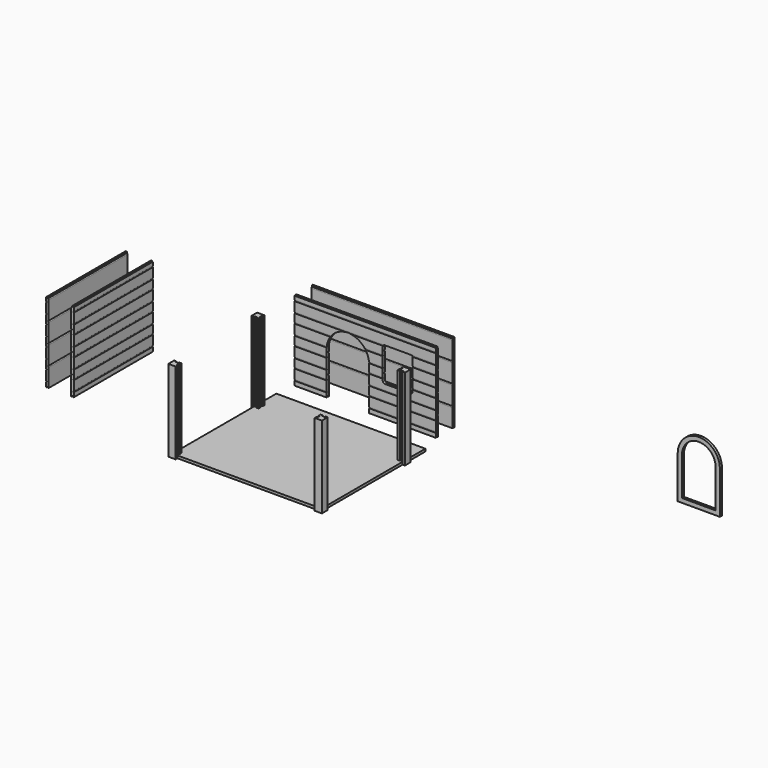
from build123d import *

# Parameters (mm, degrees)
F0_W      = 700
F0_H      = 610
F1_DEPTH  = 12
F3_DEPTH  = 384
F4_START  = -12
F4_DEPTH  = 372
F6_DEPTH  = 463.5
F8_DEPTH  = 663.5
F9_W      = 200
F9_H      = 85
F10_DEPTH = 12.5
F11_DEPTH = 12


with BuildPart() as f1:
    # F0 (on Top) → F1 (new body)
    with BuildSketch(Plane.XY):
        with Locations((0, 55)):
            Rectangle(F0_W, F0_H)
    extrude(amount=F1_DEPTH)


with BuildPart() as f3:
    # F2 (on face) → F3 (new body)
    with BuildSketch(Plane(origin=(0, 0, 0), x_dir=(1, 0, 0), z_dir=(0, 0, -1))):
        Polygon((-350, 226.75), (-350, 231.75), (-350, 250), (-331.75, 250), (-326.75, 250), (-326.75, 260.75), (-360.75, 260.75), (-360.75, 226.75), align=None)
    extrude(amount=-F3_DEPTH)

    # F2 (on face) → F4, piece 2 (join)
    with BuildSketch(Plane(origin=(0, 0, 0), x_dir=(1, 0, 0), z_dir=(0, 0, -1)).offset(F4_START)):
        Polygon((-337.5, 226.75), (-326.75, 226.75), (-326.75, 237.5), (-331.75, 237.5), (-331.75, 250), (-350, 250), (-350, 231.75), (-337.5, 231.75), align=None)
    extrude(amount=-F4_DEPTH)


with BuildPart() as f3b:
    # F2 (on face) → F3, piece 2 (new body)
    with BuildSketch(Plane(origin=(0, 0, 0), x_dir=(1, 0, 0), z_dir=(0, 0, -1))):
        Polygon((-350, -231.75), (-350, -226.75), (-360.75, -226.75), (-360.75, -260.75), (-350, -260.75), (-350, -250), align=None)
    extrude(amount=-F3_DEPTH)

    # F2 (on face) → F4, piece 4 (join)
    with BuildSketch(Plane(origin=(0, 0, 0), x_dir=(1, 0, 0), z_dir=(0, 0, -1)).offset(F4_START)):
        Polygon((-337.5, -231.75), (-350, -231.75), (-350, -250), (-350, -260.75), (-326.75, -260.75), (-326.75, -250), (-331.75, -250), (-331.75, -237.5), (-326.75, -237.5), (-326.75, -226.75), (-337.5, -226.75), align=None)
    extrude(amount=-F4_DEPTH)


with BuildPart() as f3c:
    # F2 (on face) → F3, piece 3 (new body)
    with BuildSketch(Plane(origin=(0, 0, 0), x_dir=(1, 0, 0), z_dir=(0, 0, -1))):
        Polygon((326.75, 260.75), (326.75, 250), (331.75, 250), (350, 250), (350, 231.75), (350, 226.75), (360.75, 226.75), (360.75, 260.75), align=None)
    extrude(amount=-F3_DEPTH)

    # F2 (on face) → F4 (join)
    with BuildSketch(Plane(origin=(0, 0, 0), x_dir=(1, 0, 0), z_dir=(0, 0, -1)).offset(F4_START)):
        Polygon((350, 250), (331.75, 250), (331.75, 237.5), (326.75, 237.5), (326.75, 226.75), (337.5, 226.75), (337.5, 231.75), (350, 231.75), align=None)
    extrude(amount=-F4_DEPTH)


with BuildPart() as f3d:
    # F2 (on face) → F3, piece 4 (new body)
    with BuildSketch(Plane(origin=(0, 0, 0), x_dir=(1, 0, 0), z_dir=(0, 0, -1))):
        Polygon((360.75, -226.75), (350, -226.75), (350, -231.75), (350, -250), (350, -260.75), (360.75, -260.75), align=None)
    extrude(amount=-F3_DEPTH)

    # F2 (on face) → F4, piece 3 (join)
    with BuildSketch(Plane(origin=(0, 0, 0), x_dir=(1, 0, 0), z_dir=(0, 0, -1)).offset(F4_START)):
        Polygon((326.75, -260.75), (350, -260.75), (350, -250), (350, -231.75), (337.5, -231.75), (337.5, -226.75), (326.75, -226.75), (326.75, -237.5), (331.75, -237.5), (331.75, -250), (326.75, -250), align=None)
    extrude(amount=-F4_DEPTH)


with BuildPart() as f6:
    # F5 (on face) → F6 (new body)
    with BuildSketch(Plane.XZ.offset(-231.75)):
        with BuildLine():
            Line((-836.1184597015, 267.9065500498), (-836.1184597015, 263.9065500498))
            Line((-836.1184597015, 263.9065500498), (-836.3684597015, 263.9065500498))
            ThreePointArc((-836.3684597015, 263.9065500498), (-839.1968868263, 262.7349771745), (-840.3684597015, 259.9065500498))
            Line((-840.3684597015, 259.9065500498), (-840.3684597015, 174.9065500498))
            Line((-840.3684597015, 174.9065500498), (-836.1184597015, 174.9065500498))
            Line((-836.1184597015, 174.9065500498), (-836.1184597015, 170.9065500498))
            Line((-836.1184597015, 170.9065500498), (-836.3684597015, 170.9065500498))
            ThreePointArc((-836.3684597015, 170.9065500498), (-839.1968868263, 169.7349771745), (-840.3684597015, 166.9065500498))
            Line((-840.3684597015, 166.9065500498), (-840.3684597015, 81.9065500498))
            Line((-840.3684597015, 81.9065500498), (-836.1184597015, 81.9065500498))
            Line((-836.1184597015, 81.9065500498), (-836.1184597015, 84.9065500498))
            Line((-836.1184597015, 84.9065500498), (-832.1184597015, 84.9065500498))
            Line((-832.1184597015, 84.9065500498), (-832.1184597015, 81.9065500498))
            Line((-832.1184597015, 81.9065500498), (-827.8684597015, 81.9065500498))
            Line((-827.8684597015, 81.9065500498), (-827.8684597015, 102.4065500498))
            ThreePointArc((-827.8684597015, 102.4065500498), (-830.3684597015, 104.9065500498), (-827.8684597015, 107.4065500498))
            Line((-827.8684597015, 107.4065500498), (-827.8684597015, 129.9065500498))
            Line((-827.8684597015, 129.9065500498), (-827.8684597015, 152.4065500498))
            ThreePointArc((-827.8684597015, 152.4065500498), (-830.3684597015, 154.9065500498), (-827.8684597015, 157.4065500498))
            Line((-827.8684597015, 157.4065500498), (-827.8684597015, 174.9065500498))
            Line((-827.8684597015, 174.9065500498), (-827.8684597015, 195.4065500498))
            ThreePointArc((-827.8684597015, 195.4065500498), (-830.3684597015, 197.9065500498), (-827.8684597015, 200.4065500498))
            Line((-827.8684597015, 200.4065500498), (-827.8684597015, 222.9065500498))
            Line((-827.8684597015, 222.9065500498), (-827.8684597015, 245.4065500498))
            ThreePointArc((-827.8684597015, 245.4065500498), (-830.3684597015, 247.9065500498), (-827.8684597015, 250.4065500498))
            Line((-827.8684597015, 250.4065500498), (-827.8684597015, 267.9065500498))
            Line((-827.8684597015, 267.9065500498), (-827.8684597015, 288.4065500498))
            ThreePointArc((-827.8684597015, 288.4065500498), (-830.3684597015, 290.9065500498), (-827.8684597015, 293.4065500498))
            Line((-827.8684597015, 293.4065500498), (-827.8684597015, 315.9065500498))
            Line((-827.8684597015, 315.9065500498), (-827.8684597015, 338.4065500498))
            ThreePointArc((-827.8684597015, 338.4065500498), (-830.3684597015, 340.9065500498), (-827.8684597015, 343.4065500498))
            Line((-827.8684597015, 343.4065500498), (-827.8684597015, 360.9065500498))
            Line((-827.8684597015, 360.9065500498), (-827.8684597015, 381.4065500498))
            ThreePointArc((-827.8684597015, 381.4065500498), (-830.3684597015, 383.9065500498), (-827.8684597015, 386.4065500498))
            Line((-827.8684597015, 386.4065500498), (-827.8684597015, 408.9065500498))
            Line((-827.8684597015, 408.9065500498), (-827.8684597015, 431.4065500498))
            ThreePointArc((-827.8684597015, 431.4065500498), (-830.3684597015, 433.9065500498), (-827.8684597015, 436.4065500498))
            Line((-827.8684597015, 436.4065500498), (-827.8684597015, 453.9065500498))
            Line((-827.8684597015, 453.9065500498), (-832.1184597015, 453.9065500498))
            Line((-832.1184597015, 453.9065500498), (-832.1184597015, 456.9065500498))
            Line((-832.1184597015, 456.9065500498), (-834.1184597015, 456.9065500498))
            Line((-834.1184597015, 456.9065500498), (-836.1184597015, 456.9065500498))
            Line((-836.1184597015, 456.9065500498), (-836.1184597015, 449.9065500498))
            Line((-836.1184597015, 449.9065500498), (-836.3684597015, 449.9065500498))
            ThreePointArc((-836.3684597015, 449.9065500498), (-839.1968868263, 448.7349771745), (-840.3684597015, 445.9065500498))
            Line((-840.3684597015, 445.9065500498), (-840.3684597015, 360.9065500498))
            Line((-840.3684597015, 360.9065500498), (-836.1184597015, 360.9065500498))
            Line((-836.1184597015, 360.9065500498), (-836.1184597015, 356.9065500498))
            Line((-836.1184597015, 356.9065500498), (-836.3684597015, 356.9065500498))
            ThreePointArc((-836.3684597015, 356.9065500498), (-839.1968868263, 355.7349771745), (-840.3684597015, 352.9065500498))
            Line((-840.3684597015, 352.9065500498), (-840.3684597015, 267.9065500498))
            Line((-840.3684597015, 267.9065500498), (-836.1184597015, 267.9065500498))
        make_face()
    extrude(amount=F6_DEPTH)


with BuildPart() as f6b:
    # F5 (on face) → F6, piece 2 (new body)
    with BuildSketch(Plane.XZ.offset(-231.75)):
        with BuildLine():
            Line((-949.6443090439, 170.9065500498), (-949.8943090439, 170.9065500498))
            Line((-949.8943090439, 170.9065500498), (-949.8943090439, 174.9065500498))
            Line((-949.8943090439, 174.9065500498), (-945.6443090439, 174.9065500498))
            Line((-945.6443090439, 174.9065500498), (-945.6443090439, 259.9065500498))
            ThreePointArc((-945.6443090439, 259.9065500498), (-946.8158819191, 262.7349771745), (-949.6443090439, 263.9065500498))
            Line((-949.6443090439, 263.9065500498), (-949.8943090439, 263.9065500498))
            Line((-949.8943090439, 263.9065500498), (-949.8943090439, 267.9065500498))
            Line((-949.8943090439, 267.9065500498), (-945.6443090439, 267.9065500498))
            Line((-945.6443090439, 267.9065500498), (-945.6443090439, 352.9065500498))
            ThreePointArc((-945.6443090439, 352.9065500498), (-946.8158819191, 355.7349771745), (-949.6443090439, 356.9065500498))
            Line((-949.6443090439, 356.9065500498), (-949.8943090439, 356.9065500498))
            Line((-949.8943090439, 356.9065500498), (-949.8943090439, 360.9065500498))
            Line((-949.8943090439, 360.9065500498), (-945.6443090439, 360.9065500498))
            Line((-945.6443090439, 360.9065500498), (-945.6443090439, 445.9065500498))
            ThreePointArc((-945.6443090439, 445.9065500498), (-946.8158819191, 448.7349771745), (-949.6443090439, 449.9065500498))
            Line((-949.6443090439, 449.9065500498), (-949.8943090439, 449.9065500498))
            Line((-949.8943090439, 449.9065500498), (-949.8943090439, 456.9065500498))
            Line((-949.8943090439, 456.9065500498), (-951.8943090439, 456.9065500498))
            Line((-951.8943090439, 456.9065500498), (-953.8943090439, 456.9065500498))
            Line((-953.8943090439, 456.9065500498), (-953.8943090439, 453.9065500498))
            Line((-953.8943090439, 453.9065500498), (-958.1443090439, 453.9065500498))
            Line((-958.1443090439, 453.9065500498), (-958.1443090439, 436.4065500498))
            ThreePointArc((-958.1443090439, 436.4065500498), (-955.6443090439, 433.9065500498), (-958.1443090439, 431.4065500498))
            Line((-958.1443090439, 431.4065500498), (-958.1443090439, 408.9065500498))
            Line((-958.1443090439, 408.9065500498), (-958.1443090439, 386.4065500498))
            ThreePointArc((-958.1443090439, 386.4065500498), (-955.6443090439, 383.9065500498), (-958.1443090439, 381.4065500498))
            Line((-958.1443090439, 381.4065500498), (-958.1443090439, 360.9065500498))
            Line((-958.1443090439, 360.9065500498), (-958.1443090439, 343.4065500498))
            ThreePointArc((-958.1443090439, 343.4065500498), (-955.6443090439, 340.9065500498), (-958.1443090439, 338.4065500498))
            Line((-958.1443090439, 338.4065500498), (-958.1443090439, 315.9065500498))
            Line((-958.1443090439, 315.9065500498), (-958.1443090439, 293.4065500498))
            ThreePointArc((-958.1443090439, 293.4065500498), (-955.6443090439, 290.9065500498), (-958.1443090439, 288.4065500498))
            Line((-958.1443090439, 288.4065500498), (-958.1443090439, 267.9065500498))
            Line((-958.1443090439, 267.9065500498), (-958.1443090439, 250.4065500498))
            ThreePointArc((-958.1443090439, 250.4065500498), (-955.6443090439, 247.9065500498), (-958.1443090439, 245.4065500498))
            Line((-958.1443090439, 245.4065500498), (-958.1443090439, 222.9065500498))
            Line((-958.1443090439, 222.9065500498), (-958.1443090439, 200.4065500498))
            ThreePointArc((-958.1443090439, 200.4065500498), (-955.6443090439, 197.9065500498), (-958.1443090439, 195.4065500498))
            Line((-958.1443090439, 195.4065500498), (-958.1443090439, 174.9065500498))
            Line((-958.1443090439, 174.9065500498), (-958.1443090439, 157.4065500498))
            ThreePointArc((-958.1443090439, 157.4065500498), (-955.6443090439, 154.9065500498), (-958.1443090439, 152.4065500498))
            Line((-958.1443090439, 152.4065500498), (-958.1443090439, 129.9065500498))
            Line((-958.1443090439, 129.9065500498), (-958.1443090439, 107.4065500498))
            ThreePointArc((-958.1443090439, 107.4065500498), (-955.6443090439, 104.9065500498), (-958.1443090439, 102.4065500498))
            Line((-958.1443090439, 102.4065500498), (-958.1443090439, 81.9065500498))
            Line((-958.1443090439, 81.9065500498), (-953.8943090439, 81.9065500498))
            Line((-953.8943090439, 81.9065500498), (-953.8943090439, 84.9065500498))
            Line((-953.8943090439, 84.9065500498), (-949.8943090439, 84.9065500498))
            Line((-949.8943090439, 84.9065500498), (-949.8943090439, 81.9065500498))
            Line((-949.8943090439, 81.9065500498), (-945.6443090439, 81.9065500498))
            Line((-945.6443090439, 81.9065500498), (-945.6443090439, 166.9065500498))
            ThreePointArc((-945.6443090439, 166.9065500498), (-946.8158819191, 169.7349771745), (-949.6443090439, 170.9065500498))
        make_face()
    extrude(amount=F6_DEPTH)


with BuildPart() as f8:
    # F7 (on face) → F8 (new body)
    with BuildSketch(Plane(origin=(331.75, 0, 0), x_dir=(0, -1, 0), z_dir=(-1, 0, 0))):
        with BuildLine():
            Line((-546.5363952824, 104.9655441736), (-546.7863952824, 104.9655441736))
            Line((-546.7863952824, 104.9655441736), (-546.7863952824, 108.9655441736))
            Line((-546.7863952824, 108.9655441736), (-542.5363952824, 108.9655441736))
            Line((-542.5363952824, 108.9655441736), (-542.5363952824, 193.9655441736))
            ThreePointArc((-542.5363952824, 193.9655441736), (-543.7079681576, 196.7939712984), (-546.5363952824, 197.9655441736))
            Line((-546.5363952824, 197.9655441736), (-546.7863952824, 197.9655441736))
            Line((-546.7863952824, 197.9655441736), (-546.7863952824, 201.9655441736))
            Line((-546.7863952824, 201.9655441736), (-542.5363952824, 201.9655441736))
            Line((-542.5363952824, 201.9655441736), (-542.5363952824, 286.9655441736))
            ThreePointArc((-542.5363952824, 286.9655441736), (-543.7079681576, 289.7939712984), (-546.5363952824, 290.9655441736))
            Line((-546.5363952824, 290.9655441736), (-546.7863952824, 290.9655441736))
            Line((-546.7863952824, 290.9655441736), (-546.7863952824, 294.9655441736))
            Line((-546.7863952824, 294.9655441736), (-542.5363952824, 294.9655441736))
            Line((-542.5363952824, 294.9655441736), (-542.5363952824, 379.9655441736))
            ThreePointArc((-542.5363952824, 379.9655441736), (-543.7079681576, 382.7939712984), (-546.5363952824, 383.9655441736))
            Line((-546.5363952824, 383.9655441736), (-546.7863952824, 383.9655441736))
            Line((-546.7863952824, 383.9655441736), (-546.7863952824, 390.9655441736))
            Line((-546.7863952824, 390.9655441736), (-548.7863952824, 390.9655441736))
            Line((-548.7863952824, 390.9655441736), (-550.7863952824, 390.9655441736))
            Line((-550.7863952824, 390.9655441736), (-550.7863952824, 387.9655441736))
            Line((-550.7863952824, 387.9655441736), (-555.0363952824, 387.9655441736))
            Line((-555.0363952824, 387.9655441736), (-555.0363952824, 370.4655441736))
            ThreePointArc((-555.0363952824, 370.4655441736), (-552.5363952824, 367.9655441736), (-555.0363952824, 365.4655441736))
            Line((-555.0363952824, 365.4655441736), (-555.0363952824, 342.9655441736))
            Line((-555.0363952824, 342.9655441736), (-555.0363952824, 320.4655441736))
            ThreePointArc((-555.0363952824, 320.4655441736), (-552.5363952824, 317.9655441736), (-555.0363952824, 315.4655441736))
            Line((-555.0363952824, 315.4655441736), (-555.0363952824, 294.9655441736))
            Line((-555.0363952824, 294.9655441736), (-555.0363952824, 277.4655441736))
            ThreePointArc((-555.0363952824, 277.4655441736), (-552.5363952824, 274.9655441736), (-555.0363952824, 272.4655441736))
            Line((-555.0363952824, 272.4655441736), (-555.0363952824, 249.9655441736))
            Line((-555.0363952824, 249.9655441736), (-555.0363952824, 227.4655441736))
            ThreePointArc((-555.0363952824, 227.4655441736), (-552.5363952824, 224.9655441736), (-555.0363952824, 222.4655441736))
            Line((-555.0363952824, 222.4655441736), (-555.0363952824, 201.9655441736))
            Line((-555.0363952824, 201.9655441736), (-555.0363952824, 184.4655441736))
            ThreePointArc((-555.0363952824, 184.4655441736), (-552.5363952824, 181.9655441736), (-555.0363952824, 179.4655441736))
            Line((-555.0363952824, 179.4655441736), (-555.0363952824, 156.9655441736))
            Line((-555.0363952824, 156.9655441736), (-555.0363952824, 134.4655441736))
            ThreePointArc((-555.0363952824, 134.4655441736), (-552.5363952824, 131.9655441736), (-555.0363952824, 129.4655441736))
            Line((-555.0363952824, 129.4655441736), (-555.0363952824, 108.9655441736))
            Line((-555.0363952824, 108.9655441736), (-555.0363952824, 91.4655441736))
            ThreePointArc((-555.0363952824, 91.4655441736), (-552.5363952824, 88.9655441736), (-555.0363952824, 86.4655441736))
            Line((-555.0363952824, 86.4655441736), (-555.0363952824, 63.9655441736))
            Line((-555.0363952824, 63.9655441736), (-555.0363952824, 41.4655441736))
            ThreePointArc((-555.0363952824, 41.4655441736), (-552.5363952824, 38.9655441736), (-555.0363952824, 36.4655441736))
            Line((-555.0363952824, 36.4655441736), (-555.0363952824, 15.9655441736))
            Line((-555.0363952824, 15.9655441736), (-550.7863952824, 15.9655441736))
            Line((-550.7863952824, 15.9655441736), (-550.7863952824, 18.9655441736))
            Line((-550.7863952824, 18.9655441736), (-546.7863952824, 18.9655441736))
            Line((-546.7863952824, 18.9655441736), (-546.7863952824, 15.9655441736))
            Line((-546.7863952824, 15.9655441736), (-542.5363952824, 15.9655441736))
            Line((-542.5363952824, 15.9655441736), (-542.5363952824, 100.9655441736))
            ThreePointArc((-542.5363952824, 100.9655441736), (-543.7079681576, 103.7939712984), (-546.5363952824, 104.9655441736))
        make_face()
    extrude(amount=F8_DEPTH)


with BuildPart() as f8b:
    # F7 (on face) → F8, piece 2 (new body)
    with BuildSketch(Plane(origin=(331.75, 0, 0), x_dir=(0, -1, 0), z_dir=(-1, 0, 0))):
        with BuildLine():
            Line((-453.3388936809, 108.9655441736), (-453.3388936809, 104.9655441736))
            Line((-453.3388936809, 104.9655441736), (-453.5888936809, 104.9655441736))
            ThreePointArc((-453.5888936809, 104.9655441736), (-456.4173208057, 103.7939712984), (-457.5888936809, 100.9655441736))
            Line((-457.5888936809, 100.9655441736), (-457.5888936809, 15.9655441736))
            Line((-457.5888936809, 15.9655441736), (-453.3388936809, 15.9655441736))
            Line((-453.3388936809, 15.9655441736), (-453.3388936809, 18.9655441736))
            Line((-453.3388936809, 18.9655441736), (-449.3388936809, 18.9655441736))
            Line((-449.3388936809, 18.9655441736), (-449.3388936809, 15.9655441736))
            Line((-449.3388936809, 15.9655441736), (-445.0888936809, 15.9655441736))
            Line((-445.0888936809, 15.9655441736), (-445.0888936809, 36.4655441736))
            ThreePointArc((-445.0888936809, 36.4655441736), (-447.5888936809, 38.9655441736), (-445.0888936809, 41.4655441736))
            Line((-445.0888936809, 41.4655441736), (-445.0888936809, 63.9655441736))
            Line((-445.0888936809, 63.9655441736), (-445.0888936809, 86.4655441736))
            ThreePointArc((-445.0888936809, 86.4655441736), (-447.5888936809, 88.9655441736), (-445.0888936809, 91.4655441736))
            Line((-445.0888936809, 91.4655441736), (-445.0888936809, 108.9655441736))
            Line((-445.0888936809, 108.9655441737), (-445.0888936809, 129.4655441737))
            ThreePointArc((-445.0888936809, 129.4655441737), (-447.5888936809, 131.9655441737), (-445.0888936809, 134.4655441737))
            Line((-445.0888936809, 134.4655441737), (-445.0888936809, 156.9655441737))
            Line((-445.0888936809, 156.9655441737), (-445.0888936809, 179.4655441737))
            ThreePointArc((-445.0888936809, 179.4655441737), (-447.5888936809, 181.9655441737), (-445.0888936809, 184.4655441737))
            Line((-445.0888936809, 184.4655441737), (-445.0888936809, 201.9655441737))
            Line((-445.0888936809, 201.9655441739), (-445.0888936809, 222.4655441739))
            ThreePointArc((-445.0888936809, 222.4655441739), (-447.5888936809, 224.9655441739), (-445.0888936809, 227.4655441739))
            Line((-445.0888936809, 227.4655441739), (-445.0888936809, 249.9655441739))
            Line((-445.0888936809, 249.9655441739), (-445.0888936809, 272.4655441739))
            ThreePointArc((-445.0888936809, 272.4655441739), (-447.5888936809, 274.9655441739), (-445.0888936809, 277.4655441739))
            Line((-445.0888936809, 277.4655441739), (-445.0888936809, 294.9655441739))
            Line((-445.0888936809, 294.965544174), (-445.0888936809, 315.465544174))
            ThreePointArc((-445.0888936809, 315.465544174), (-447.5888936809, 317.965544174), (-445.0888936809, 320.465544174))
            Line((-445.0888936809, 320.465544174), (-445.0888936809, 342.965544174))
            Line((-445.0888936809, 342.965544174), (-445.0888936809, 365.465544174))
            ThreePointArc((-445.0888936809, 365.465544174), (-447.5888936809, 367.965544174), (-445.0888936809, 370.465544174))
            Line((-445.0888936809, 370.465544174), (-445.0888936809, 387.965544174))
            Line((-445.0888936809, 387.965544174), (-449.3388936809, 387.965544174))
            Line((-449.3388936809, 387.965544174), (-449.3388936809, 390.965544174))
            Line((-449.3388936809, 390.965544174), (-451.3388936809, 390.965544174))
            Line((-451.3388936809, 390.965544174), (-453.3388936809, 390.965544174))
            Line((-453.3388936809, 390.965544174), (-453.3388936809, 383.965544174))
            Line((-453.3388936809, 383.965544174), (-453.5888936809, 383.965544174))
            ThreePointArc((-453.5888936809, 383.965544174), (-456.4173208057, 382.7939712987), (-457.5888936809, 379.965544174))
            Line((-457.5888936809, 379.965544174), (-457.5888936809, 294.965544174))
            Line((-457.5888936809, 294.965544174), (-453.3388936809, 294.965544174))
            Line((-453.3388936809, 294.965544174), (-453.3388936809, 290.9655441739))
            Line((-453.3388936809, 290.9655441739), (-453.5888936809, 290.9655441739))
            ThreePointArc((-453.5888936809, 290.9655441739), (-456.4173208057, 289.7939712986), (-457.5888936809, 286.9655441739))
            Line((-457.5888936809, 286.9655441739), (-457.5888936809, 201.9655441739))
            Line((-457.5888936809, 201.9655441739), (-453.3388936809, 201.9655441739))
            Line((-453.3388936809, 201.9655441739), (-453.3388936809, 197.9655441737))
            Line((-453.3388936809, 197.9655441737), (-453.5888936809, 197.9655441737))
            ThreePointArc((-453.5888936809, 197.9655441737), (-456.4173208057, 196.7939712985), (-457.5888936809, 193.9655441737))
            Line((-457.5888936809, 193.9655441737), (-457.5888936809, 108.9655441737))
            Line((-457.5888936809, 108.9655441737), (-453.3388936809, 108.9655441736))
        make_face()
    extrude(amount=F8_DEPTH)

    # F9 (on face) → F10 (cut)
    with BuildSketch(Plane(origin=(0, 457.5888936809, 0), x_dir=(-1, 0, 0), z_dir=(0, 1, 0))):
        with BuildLine():
            ThreePointArc((-81.75, 310.965544174), (-84.6789321881, 318.0366119858), (-91.75, 320.965544174))
            Line((-91.75, 320.965544174), (-211.75, 320.965544174))
            ThreePointArc((-211.75, 320.965544174), (-218.8210678119, 318.0366119858), (-221.75, 310.965544174))
            Line((-221.75, 310.965544174), (-221.75, 170.965544174))
            ThreePointArc((-221.75, 170.965544174), (-218.8210678119, 163.8944763621), (-211.75, 160.965544174))
            Line((-211.75, 160.965544174), (-91.75, 160.965544174))
            ThreePointArc((-91.75, 160.965544174), (-84.6789321881, 163.8944763621), (-81.75, 170.965544174))
            Line((-81.75, 170.965544174), (-81.75, 310.965544174))
        make_face()
        with BuildLine():
            Line((-18.25, 215.9655441736), (-18.25, 100.9655441736))
            Line((-18.25, 100.9655441736), (181.75, 100.9655441736))
            Line((181.75, 100.9655441736), (181.75, 215.9655441736))
            ThreePointArc((181.75, 215.9655441736), (152.4606781187, 286.6762222923), (81.75, 315.9655441736))
            ThreePointArc((81.75, 315.9655441736), (11.0393218813, 286.6762222923), (-18.25, 215.9655441736))
        make_face()
        with Locations((81.75, 58.4655441736)):
            Rectangle(F9_W, F9_H)
    extrude(amount=-F10_DEPTH, mode=Mode.SUBTRACT)


with BuildPart() as f11:
    # F9 (on face) → F11 (new body)
    with BuildSketch(Plane(origin=(0, 457.5888936809, 0), x_dir=(-1, 0, 0), z_dir=(0, 1, 0))):
        with BuildLine():
            Line((-1664.8818445206, 321.8039312214), (-1664.8818445206, 122.8039312214))
            Line((-1664.8818445206, 122.8039312214), (-1466.8818445206, 122.8039312214))
            Line((-1466.8818445206, 122.8039312214), (-1466.8818445206, 321.8039312214))
            ThreePointArc((-1466.8818445206, 321.8039312214), (-1495.8782731831, 391.8075025588), (-1565.8818445206, 420.8039312214))
            ThreePointArc((-1565.8818445206, 420.8039312214), (-1635.885415858, 391.8075025588), (-1664.8818445206, 321.8039312214))
        make_face()
        with BuildLine():
            Line((-1486.8818445206, 142.8039312214), (-1644.8818445206, 142.8039312214))
            Line((-1644.8818445206, 142.8039312214), (-1644.8818445206, 321.8039312214))
            ThreePointArc((-1644.8818445206, 321.8039312214), (-1622.0957218108, 377.3106875669), (-1566.8818445206, 400.7976018539))
            ThreePointArc((-1566.8818445206, 400.7976018539), (-1510.3750881751, 378.0178085116), (-1486.8818445206, 321.8039312214))
            Line((-1486.8818445206, 321.8039312214), (-1486.8818445206, 142.8039312214))
        make_face(mode=Mode.SUBTRACT)
    extrude(amount=-F11_DEPTH)


solid = Compound([f1.part, f3.part, f3b.part, f3c.part, f3d.part, f6.part, f6b.part, f8.part, f8b.part, f11.part])
